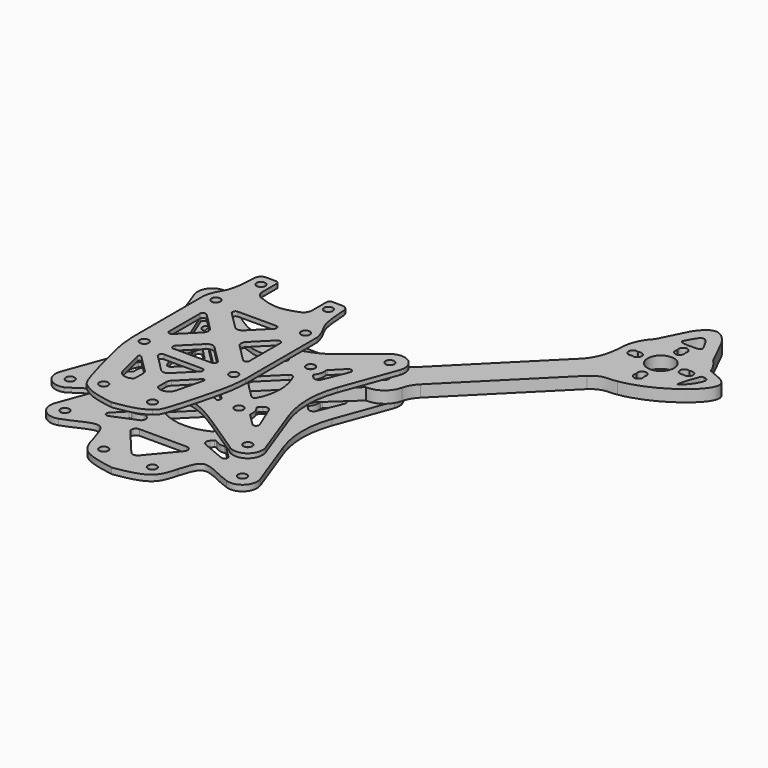
from build123d import *

# Parameters (mm, degrees)
F0_R     = 1.5
F2_DEPTH = 2
F4_START = 3
F1_R     = 1.5
F1_R_2   = 4.5
F4_DEPTH = 4
F7_START = 20
F6_R     = 1.5
F7_DEPTH = 1.5
F8_START = 9
F5_R     = 1.5
F8_DEPTH = 1.5


with BuildPart() as f2:
    # F0 (on Top) → F2 (new body)
    with BuildSketch(Plane.XY):
        with BuildLine():
            add(Edge.make_bspline(
                [(-28.6583371689, 34.989895508), (-15.5486081514, 28.1029236725), (-15.2531134537, 20.3288752095), (-15.0275822655, 35.7869570093)],
                knots=[0, 0, 0, 0, 13.3992828802, 13.3992828802, 13.3992828802, 13.3992828802], degree=3))
            ThreePointArc((-28.6583371689, 34.989895508), (-33.8221162144, 33.7485690999), (-34.9557615497, 28.560086322))
            Line((-34.9557615497, 28.560086322), (-28.2756954338, 10.3133747837))
            ThreePointArc((-28.2756954338, 10.3133747837), (-26.4471685044, -7.1088e-06), (-28.2756201348, -10.3134023513))
            Line((-28.2756201348, -10.3134023513), (-34.9643155344, -28.58409813))
            ThreePointArc((-34.9643155344, -28.58409813), (-33.8042341838, -33.7667341911), (-28.6341939914, -34.9817196608))
            add(Edge.make_bspline(
                [(-28.6341939914, -34.9817196608), (-24.495487875, -33.6930387827), (-16.3607874703, -27.7449542077), (-15.1366587225, -35.7631260416), (-14.33, -37.7577804035)],
                knots=[0, 0, 0, 0, 0.5615113554, 1, 1, 1, 1], degree=3))
            add(Edge.make_bspline(
                [(-14.33, -37.7577804035), (-13.6367446794, -40.3263257967), (-12.088150953, -46.0639424644), (-4.3010614265, -47.3817279873), (0, -48.1095835567)],
                knots=[0, 0, 0, 0, 0.447667654, 1, 1, 1, 1], degree=3))
            add(Edge.make_bspline(
                [(14.33, -37.7577804035), (13.6367446794, -40.3263257967), (12.088150953, -46.0639424644), (4.3010614265, -47.3817279873), (0, -48.1095835567)],
                knots=[0, 0, 0, 0, 0.447667654, 1, 1, 1, 1], degree=3))
            add(Edge.make_bspline(
                [(28.6583371689, -34.9898955092), (24.5097770544, -33.6967999), (16.3601661117, -27.7422129401), (15.1363049951, -35.7630085829), (14.33, -37.7577804035)],
                knots=[0, 0, 0, 0, 0.561784833, 1, 1, 1, 1], degree=3))
            ThreePointArc((28.6583371689, -34.9898955092), (33.8221162144, -33.748569101), (34.9557615497, -28.5600863232))
            Line((34.9557615497, -28.5600863232), (28.2756954338, -10.3133747849))
            ThreePointArc((28.2756954338, -10.3133747849), (26.4471685044, 7.1077e-06), (28.2756201348, 10.3134023502))
            Line((28.2756201348, 10.3134023502), (34.9643155344, 28.5840981288))
            ThreePointArc((34.9643155344, 28.5840981288), (33.8042341838, 33.76673419), (28.6341939914, 34.9817196596))
            add(Edge.make_bspline(
                [(15.0274820378, 35.7867377887), (15.2513136358, 20.3289797995), (15.5248044507, 28.1031931102), (28.6341939914, 34.9817196596)],
                knots=[0.5359060708, 0.5359060708, 0.5359060708, 0.5359060708, 13.9139411757, 13.9139411757, 13.9139411757, 13.9139411757], degree=3))
            ThreePointArc((15.0274820378, 35.7867377887), (14.4316299327, 37.1821951546), (13.0276916813, 37.7577804023))
            Line((13.0276916813, 37.7577804023), (-13.0277950954, 37.7577804023))
            ThreePointArc((-13.0277950954, 37.7577804023), (-14.4316552711, 37.1822721036), (-15.0275822655, 35.7869570093))
        make_face()
        with Locations((-30.25, -30.2500000006)):
            Circle(F0_R, mode=Mode.SUBTRACT)
        with Locations((-8.2733329443, -41.1618490551)):
            Circle(F0_R, mode=Mode.SUBTRACT)
        with BuildLine():
            ThreePointArc((-23.8517090122, -20.3161751069), (-25.1141961389, -20.4406647854), (-25.4828700073, -19.2268068843))
            Line((-25.4828700073, -19.2268068843), (-22.1833207357, -11.2506887671))
            ThreePointArc((-22.1833207357, -11.2506887671), (-21.0902108457, -10.3529698728), (-19.736579243, -10.7634207575))
            Line((-19.736579243, -10.7634207575), (-18.8553009264, -11.6446990741))
            ThreePointArc((-18.8553009264, -11.6446990741), (-18.7090370991, -11.9847340093), (-18.8367068235, -12.33217797))
            Line((-18.8367068235, -12.33217797), (-18.8542943682, -12.3517786311))
            ThreePointArc((-18.8542943682, -12.3517786311), (-19.6877326512, -13.9472514003), (-19.8489637612, -15.7400584892))
            Line((-19.8489637612, -15.7400584892), (-19.8303976916, -15.8549305034))
            ThreePointArc((-19.8303976916, -15.8549305034), (-19.8571321349, -16.2052315209), (-20.0404595752, -16.5049256699))
            Line((-20.0404595752, -16.5049256699), (-23.8517090122, -20.3161751069))
        make_face(mode=Mode.SUBTRACT)
        with BuildLine():
            Line((-11.2506887665, -22.1833207364), (-19.2268068836, -25.482870008))
            ThreePointArc((-19.2268068836, -25.482870008), (-20.4406647847, -25.1141961396), (-20.3161751062, -23.8517090128))
            Line((-20.3161751062, -23.8517090128), (-16.5049256693, -20.0404595759))
            ThreePointArc((-16.5049256693, -20.0404595759), (-16.2052315202, -19.8571321356), (-15.8549305027, -19.8303976923))
            Line((-15.8549305027, -19.8303976923), (-15.7400584885, -19.8489637619))
            ThreePointArc((-15.7400584885, -19.8489637619), (-13.9472513996, -19.6877326519), (-12.3517786304, -18.8542943689))
            Line((-12.3517786304, -18.8542943689), (-12.3321779693, -18.8367068242))
            ThreePointArc((-12.3321779693, -18.8367068242), (-11.9847340086, -18.7090370997), (-11.6446990734, -18.8553009271))
            Line((-11.6446990734, -18.8553009271), (-10.7634207569, -19.7365792436))
            ThreePointArc((-10.7634207569, -19.7365792436), (-10.3529698721, -21.0902108464), (-11.2506887665, -22.1833207364))
        make_face(mode=Mode.SUBTRACT)
        with Locations((-15.25, -15.2500000006)):
            Circle(F0_R, mode=Mode.SUBTRACT)
        with BuildLine():
            ThreePointArc((-7.7892382513, -15.2383616248), (-8.2896410828, -14.5053634666), (-8.0071487762, -13.6640030263))
            Line((-8.0071487762, -13.6640030263), (-1.4142135624, -7.0710678125))
            ThreePointArc((-1.4142135624, -7.0710678125), (0, -6.4852813748), (1.4142135624, -7.0710678125))
            Line((1.4142135624, -7.0710678125), (8.0039929944, -13.6608472445))
            ThreePointArc((8.0039929944, -13.6608472445), (8.287442711, -14.5050591849), (7.7853439372, -15.2405415869))
            Line((7.7853439372, -15.2405415869), (7.7684472975, -15.2500000006))
            ThreePointArc((7.7684472975, -15.2500000006), (0, -17.1146508417), (-7.7684472975, -15.2500000006))
            Line((-7.7684472975, -15.2500000006), (-7.7892382513, -15.2383616248))
        make_face(mode=Mode.SUBTRACT)
        with Locations((8.2733329443, -41.1618490551)):
            Circle(F0_R, mode=Mode.SUBTRACT)
        with BuildLine():
            Line((-1.3419338656, -38.0910861377), (-9.1892168108, -28.7161126104))
            ThreePointArc((-9.1892168108, -28.7161126104), (-9.3980668278, -27.118570832), (-8.0389877832, -26.2533181443))
            Line((-8.0389877832, -26.2533181443), (8.0389877833, -26.2533181443))
            ThreePointArc((8.0389877833, -26.2533181443), (9.398066828, -27.118570832), (9.189216811, -28.7161126104))
            Line((9.189216811, -28.7161126104), (1.3419338656, -38.0910861377))
            ThreePointArc((1.3419338656, -38.0910861377), (0, -38.7178259272), (-1.3419338656, -38.0910861377))
        make_face(mode=Mode.SUBTRACT)
        with Locations((30.25, -30.2500000006)):
            Circle(F0_R, mode=Mode.SUBTRACT)
        with BuildLine():
            ThreePointArc((20.3161751064, -23.8517090128), (20.4406647849, -25.1141961396), (19.2268068838, -25.482870008))
            Line((19.2268068838, -25.482870008), (11.2506887667, -22.1833207364))
            ThreePointArc((11.2506887667, -22.1833207364), (10.3529698723, -21.0902108464), (10.7634207571, -19.7365792436))
            Line((10.7634207571, -19.7365792436), (11.6446990736, -18.8553009271))
            ThreePointArc((11.6446990736, -18.8553009271), (11.9847340088, -18.7090370997), (12.3321779695, -18.8367068242))
            Line((12.3321779695, -18.8367068242), (12.3517786306, -18.8542943689))
            ThreePointArc((12.3517786306, -18.8542943689), (13.9472513998, -19.6877326519), (15.7400584887, -19.8489637619))
            Line((15.7400584887, -19.8489637619), (15.8549305029, -19.8303976923))
            ThreePointArc((15.8549305029, -19.8303976923), (16.2052315204, -19.8571321356), (16.5049256694, -20.0404595759))
            Line((16.5049256694, -20.0404595759), (20.3161751064, -23.8517090128))
        make_face(mode=Mode.SUBTRACT)
        with Locations((15.25, -15.2500000006)):
            Circle(F0_R, mode=Mode.SUBTRACT)
        with BuildLine():
            ThreePointArc((19.7365792431, -10.7634207575), (21.0902108459, -10.3529698728), (22.1833207359, -11.2506887671))
            Line((22.1833207359, -11.2506887671), (25.4828700075, -19.2268068842))
            ThreePointArc((25.4828700075, -19.2268068842), (25.1141961391, -20.4406647853), (23.8517090123, -20.3161751069))
            Line((23.8517090123, -20.3161751069), (20.0404595754, -16.5049256699))
            ThreePointArc((20.0404595754, -16.5049256699), (19.8571321351, -16.2052315209), (19.8303976918, -15.8549305033))
            Line((19.8303976918, -15.8549305033), (19.8489637614, -15.7400584892))
            ThreePointArc((19.8489637614, -15.7400584892), (19.6877326514, -13.9472514003), (18.8542943684, -12.3517786311))
            Line((18.8542943684, -12.3517786311), (18.8367068237, -12.33217797))
            ThreePointArc((18.8367068237, -12.33217797), (18.7090370992, -11.9847340093), (18.8553009266, -11.6446990741))
            Line((18.8553009266, -11.6446990741), (19.7365792431, -10.7634207575))
        make_face(mode=Mode.SUBTRACT)
        with BuildLine():
            ThreePointArc((-18.8367068237, 12.3321779688), (-18.7090370992, 11.9847340081), (-18.8553009266, 11.6446990729))
            Line((-18.8553009266, 11.6446990729), (-19.7365318181, 10.7634681813))
            ThreePointArc((-19.7365318181, 10.7634681813), (-21.0901735727, 10.3530193183), (-22.1832812244, 11.250755321))
            Line((-22.1832812244, 11.250755321), (-25.4825410679, 19.2264854211))
            ThreePointArc((-25.4825410679, 19.2264854211), (-25.1138561851, 20.4403344014), (-23.851374797, 20.3158408904))
            Line((-23.851374797, 20.3158408904), (-20.0404595754, 16.5049256687))
            ThreePointArc((-20.0404595754, 16.5049256687), (-19.8571321351, 16.2052315197), (-19.8303976918, 15.8549305022))
            Line((-19.8303976918, 15.8549305022), (-19.8489637614, 15.740058488))
            ThreePointArc((-19.8489637614, 15.740058488), (-19.6877326514, 13.9472513991), (-18.8542943684, 12.3517786299))
            Line((-18.8542943684, 12.3517786299), (-18.8367068237, 12.3321779688))
        make_face(mode=Mode.SUBTRACT)
        with BuildLine():
            ThreePointArc((-13.6608472446, -8.003992994), (-14.505059185, -8.2874427105), (-15.2405415869, -7.7853439367))
            Line((-15.2405415869, -7.7853439367), (-15.25, -7.7684472983))
            ThreePointArc((-15.25, -7.7684472983), (-17.1146508411, -6e-10), (-15.25, 7.7684472971))
            Line((-15.25, 7.7684472971), (-15.2405415859, 7.7853439372))
            ThreePointArc((-15.2405415859, 7.7853439372), (-14.505059184, 8.2874427111), (-13.6608472436, 8.0039929945))
            Line((-13.6608472436, 8.0039929945), (-7.0710678122, 1.4142135631))
            ThreePointArc((-7.0710678122, 1.4142135631), (-6.4852813746, 7e-10), (-7.0710678122, -1.4142135616))
            Line((-7.0710678122, -1.4142135616), (-13.6608472446, -8.003992994))
        make_face(mode=Mode.SUBTRACT)
        with Locations((-15.25, 15.2499999994)):
            Circle(F0_R, mode=Mode.SUBTRACT)
        with BuildLine():
            ThreePointArc((7.7853439372, 15.2405415857), (8.287442711, 14.5050591838), (8.0039929944, 13.6608472433))
            Line((8.0039929944, 13.6608472433), (1.4142135624, 7.0710678113))
            ThreePointArc((1.4142135624, 7.0710678113), (0, 6.4852813737), (-1.4142135624, 7.0710678113))
            Line((-1.4142135624, 7.0710678113), (-8.0039929944, 13.6608472433))
            ThreePointArc((-8.0039929944, 13.6608472433), (-8.287442711, 14.5050591838), (-7.7853439372, 15.2405415857))
            Line((-7.7853439372, 15.2405415857), (-7.7684472975, 15.2499999994))
            ThreePointArc((-7.7684472975, 15.2499999994), (0, 17.1146508406), (7.7684472975, 15.2499999994))
            Line((7.7684472975, 15.2499999994), (7.7853439372, 15.2405415857))
        make_face(mode=Mode.SUBTRACT)
        with Locations((-30.25, 30.2499999994)):
            Circle(F0_R, mode=Mode.SUBTRACT)
        with BuildLine():
            ThreePointArc((-7.7684472975, 20.1190513336), (-9.4080907996, 20.7386520685), (-8.9382902045, 22.4273270773))
            Line((-8.9382902045, 22.4273270773), (-1.06072927, 27.355528746))
            ThreePointArc((-1.06072927, 27.355528746), (0, 27.6599894761), (1.0607292699, 27.355528746))
            Line((1.0607292699, 27.355528746), (8.9382902045, 22.4273270773))
            ThreePointArc((8.9382902045, 22.4273270773), (9.4121452662, 20.7467816187), (7.7853439372, 20.1125189809))
            ThreePointArc((7.7853439372, 20.1125189809), (0.0090577048, 21.5667549236), (-7.7684472975, 20.1190513336))
        make_face(mode=Mode.SUBTRACT)
        with Locations((-11.5, 29.7577804023)):
            Circle(F0_R, mode=Mode.SUBTRACT)
        with BuildLine():
            Line((7.0710678124, 1.4142135624), (13.6608472439, 8.0039929938))
            ThreePointArc((13.6608472439, 8.0039929938), (14.5050591843, 8.2874427104), (15.2405415863, 7.7853439366))
            Line((15.2405415863, 7.7853439366), (15.25, 7.7684472971))
            ThreePointArc((15.25, 7.7684472971), (17.1146508411, -6e-10), (15.25, -7.7684472983))
            Line((15.25, -7.7684472983), (15.2405415867, -7.7853439371))
            ThreePointArc((15.2405415867, -7.7853439371), (14.5050591848, -8.2874427109), (13.6608472444, -8.0039929943))
            Line((13.6608472444, -8.0039929943), (7.0710678124, -1.4142135624))
            ThreePointArc((7.0710678124, -1.4142135624), (6.4852813748, 0), (7.0710678124, 1.4142135624))
        make_face(mode=Mode.SUBTRACT)
        with Locations((15.25, 15.2499999994)):
            Circle(F0_R, mode=Mode.SUBTRACT)
        with BuildLine():
            Line((19.8247048971, 15.785759925), (19.8053184489, 15.9004963368))
            ThreePointArc((19.8053184489, 15.9004963368), (19.8295490283, 16.2509794496), (20.0107302331, 16.5519759685))
            Line((20.0107302331, 16.5519759685), (23.8084562188, 20.4043695836))
            ThreePointArc((23.8084562188, 20.4043695836), (25.0693920791, 20.5382911332), (25.4479247727, 19.3280815542))
            Line((25.4479247727, 19.3280815542), (22.2099579078, 11.3050038785))
            ThreePointArc((22.2099579078, 11.3050038785), (21.1235499455, 10.3976310998), (19.7659136105, 10.7981697397))
            Line((19.7659136105, 10.7981697397), (18.8636878016, 11.6875924575))
            ThreePointArc((18.8636878016, 11.6875924575), (18.7150078324, 12.0262851571), (18.8397994936, 12.37448843))
            Line((18.8397994936, 12.37448843), (18.8575858105, 12.3946446988))
            ThreePointArc((18.8575858105, 12.3946446988), (19.6770217108, 13.9944130467), (19.8247048971, 15.785759925))
        make_face(mode=Mode.SUBTRACT)
        with Locations((11.5, 29.7577804023)):
            Circle(F0_R, mode=Mode.SUBTRACT)
        with Locations((30.25, 30.2499999994)):
            Circle(F0_R, mode=Mode.SUBTRACT)
    extrude(amount=F2_DEPTH)


with BuildPart() as f4:
    # F1 (on Top) → F4 (new body)
    with BuildSketch(Plane.XY.offset(F4_START)):
        with BuildLine():
            add(Edge.make_bspline(
                [(77.2593953395, 101.7986398484), (78.7593953395, 104.1420138718), (82.5093953395, 107.8579861282), (86.2593953395, 104.1420138718), (87.7593953395, 101.7986398484)],
                knots=[0, 0, 0, 0, 0.5, 1, 1, 1, 1], degree=3))
            Line((77.2593953395, 101.7986398484), (72.6099004029, 92.3994949366))
            ThreePointArc((72.6099004029, 92.3994949366), (69.5750818843, 87.8575680531), (68.5093953395, 82.5))
            add(Edge.make_bspline(
                [(64.6217106464, 71.6833831188), (67.2594552161, 74.6181810973), (68.3412179351, 78.679420054), (68.5093953395, 82.5)],
                knots=[0, 0, 0, 0, 11.4940546817, 11.4940546817, 11.4940546817, 11.4940546817], degree=3))
            Line((64.6217106464, 71.6833831188), (33.0976358255, 40.1593082979))
            ThreePointArc((33.0976358255, 40.1593082979), (30.9505970873, 38.5267023061), (28.4453264856, 37.5273040471))
            ThreePointArc((28.4453264856, 37.5273040471), (24.6916297412, 35.2749364416), (22.834774137, 31.3106601718))
            Line((22.834774137, 31.3106601718), (13.6185183249, 19.9730840161))
            ThreePointArc((13.6185183249, 19.9730840161), (11.3998018999, 18.428606374), (10.3093393921, 15.9549440526))
            Line((10.3093393921, 15.9549440526), (6.3693953395, 12.015))
            Line((6.3693953395, 12.015), (0.0093953395, 5.655))
            Line((0.0093953395, 5.655), (0.0093953395, 0))
            Line((0.0093953395, 0), (5.6643953395, 0))
            Line((5.6643953395, 0), (12.0243953395, 6.36))
            Line((12.0243953395, 6.36), (15.964339392, 10.2999440526))
            ThreePointArc((15.964339392, 10.2999440526), (18.4380017135, 11.3904065604), (19.9824793556, 13.6091229854))
            Line((19.9824793556, 13.6091229854), (29.8420821702, 22.7616190189))
            ThreePointArc((29.8420821702, 22.7616190189), (34.7107235952, 24.2138027898), (37.5366993865, 28.4359311461))
            ThreePointArc((37.5366993865, 28.4359311461), (38.5360976455, 30.9412017478), (40.1687036374, 33.0882404861))
            Line((40.1687036374, 33.0882404861), (71.6788756749, 64.5984125236))
            add(Edge.make_bspline(
                [(71.6788756749, 64.5984125236), (75.2138197422, 67.773707211), (77.5027647614, 66.6008293629), (80.0291356677, 67.1997283697)],
                knots=[0, 0, 0, 0, 8.7460668919, 8.7460668919, 8.7460668919, 8.7460668919], degree=3))
            add(Edge.make_bspline(
                [(95.6294447875, 87.3851102834), (98.5490253606, 86.1806662064), (109.349192454, 82.9975524374), (90.7150401258, 68.8518105531), (80.0291356677, 67.1997283697)],
                knots=[0, 0, 0, 0, 0.3577567319, 1, 1, 1, 1], degree=3))
            ThreePointArc((95.6294447875, 87.3851102834), (94.2890756952, 90.0656546787), (92.4088902761, 92.3994949366))
            Line((92.4088902761, 92.3994949366), (87.7593953395, 101.7986398484))
        make_face()
        with Locations((15.2593953395, 15.25)):
            Circle(F1_R, mode=Mode.SUBTRACT)
        with Locations((30.2593953395, 30.25)):
            Circle(F1_R, mode=Mode.SUBTRACT)
        with BuildLine():
            ThreePointArc((83.8084334452, 73.75), (82.5093953395, 71.5), (81.2103572338, 73.75))
            ThreePointArc((81.2103572338, 73.75), (82.5093953395, 76), (83.8084334452, 73.75))
        make_face(mode=Mode.SUBTRACT)
        with BuildLine():
            add(Edge.make_bspline(
                [(96.4851732404, 83.323184101), (95.8861932158, 83.3624526858), (95.6489634201, 83.406211956), (92.4634486437, 74.1656348109), (94.1752940416, 76.0721862316)],
                knots=[0, 0, 0, 0, 0.3095337058, 1, 1, 1, 1], degree=3))
            add(Edge.make_bspline(
                [(96.4851732404, 83.323184101), (97.1968024969, 83.2540988922), (99.2072247022, 82.7650440123), (96.5406354296, 78.1400697337), (94.1752940416, 76.0721862316)],
                knots=[0, 0, 0, 0, 0.324824519, 1, 1, 1, 1], degree=3))
        make_face(mode=Mode.SUBTRACT)
        with BuildLine():
            ThreePointArc((73.7593953395, 83.7990381057), (76.0093953395, 82.5), (73.7593953395, 81.2009618943))
            ThreePointArc((73.7593953395, 81.2009618943), (71.5093953395, 82.5), (73.7593953395, 83.7990381057))
        make_face(mode=Mode.SUBTRACT)
        with Locations((82.5093953395, 82.5)):
            Circle(F1_R_2, mode=Mode.SUBTRACT)
        with BuildLine():
            ThreePointArc((91.2593953395, 81.2009618943), (89.0093953395, 82.5), (91.2593953395, 83.7990381057))
            ThreePointArc((91.2593953395, 83.7990381057), (93.5093953395, 82.5), (91.2593953395, 81.2009618943))
        make_face(mode=Mode.SUBTRACT)
        with BuildLine():
            ThreePointArc((83.8084334452, 91.25), (82.5093953395, 89), (81.2103572338, 91.25))
            ThreePointArc((81.2103572338, 91.25), (82.5093953395, 93.5), (83.8084334452, 91.25))
        make_face(mode=Mode.SUBTRACT)
        with BuildLine():
            add(Edge.make_bspline(
                [(79.0163052703, 96.0572239698), (79.135660109, 95.064372308), (82.5093953395, 95.064372308), (85.88313057, 95.064372308), (86.0024854087, 96.0572239698)],
                knots=[0, 0, 0, 0, 0.5, 1, 1, 1, 1], degree=3))
            add(Edge.make_bspline(
                [(79.0163052703, 96.0572239698), (80.1806686267, 98.4065499989), (82.5093953395, 103.1052020569), (84.8381220523, 98.4065499989), (86.0024854087, 96.0572239698)],
                knots=[0, 0, 0, 0, 0.5, 1, 1, 1, 1], degree=3))
        make_face(mode=Mode.SUBTRACT)
    extrude(amount=F4_DEPTH)


with BuildPart() as f7:
    # F6 (on Top) → F7 (new body)
    with BuildSketch(Plane.XY.offset(F7_START)):
        with BuildLine():
            add(Edge.make_bspline(
                [(-19.25, -15.2218541075), (-19.0684905374, -19.7268529833), (-17.9623264747, -24.6907042809), (-13.2785718821, -43.084666195), (-11.6053951728, -44.1968771124), (-11.0003547743, -44.5749795424)],
                knots=[0, 0, 0, 0, 0.3683029461, 0.8298524693, 1, 1, 1, 1], degree=3))
            add(Edge.make_bspline(
                [(-11.0003547743, -44.5749795424), (-7.8986920416, -46.9837644324), (-3.9995196275, -47.3454079802), (0, -48.1093942399)],
                knots=[0, 0, 0, 0, 11.5542153526, 11.5542153526, 11.5542153526, 11.5542153526], degree=3))
            add(Edge.make_bspline(
                [(11.0003547743, -44.5749795424), (7.8986920416, -46.9837644324), (3.9995196275, -47.3454079802), (0, -48.1093942399)],
                knots=[0, 0, 0, 0, 11.5542153526, 11.5542153526, 11.5542153526, 11.5542153526], degree=3))
            add(Edge.make_bspline(
                [(19.25, -15.2218541075), (19.0667337669, -19.7267716154), (17.9562925595, -24.6902276301), (13.2790290127, -43.0847539077), (11.6055152346, -44.1969091306), (11.0003547743, -44.5749795424)],
                knots=[0, 0, 0, 0, 0.368314136, 0.829851714, 1, 1, 1, 1], degree=3))
            Line((19.25, -15.2218541075), (19.25, 15.2781458925))
            add(Edge.make_bspline(
                [(15.0790967662, 31.8597836794), (15.7273210805, 18.4148469189), (17.670676786, 22.4575338068), (19.25, 15.2781458925)],
                knots=[0.8128411452, 0.8128411452, 0.8128411452, 0.8128411452, 18.97635654, 18.97635654, 18.97635654, 18.97635654], degree=3))
            ThreePointArc((15.0790967662, 31.8597836794), (14.4611582834, 33.211334576), (13.0814172406, 33.7634690247))
            add(Edge.make_bspline(
                [(9.5020394819, 33.7713114856), (10.6902314797, 33.7688881845), (11.9558724743, 33.7634690247), (13.0814172406, 33.7634690247)],
                knots=[1.0243447025, 1.0243447025, 1.0243447025, 1.0243447025, 4.5814260604, 4.5814260604, 4.5814260604, 4.5814260604], degree=3))
            ThreePointArc((9.5020394819, 33.7713114856), (8.7936146526, 33.479141045), (8.5, 32.7713135654))
            add(Edge.make_bspline(
                [(8.5, 32.285449478), (8.5, 32.4472244474), (8.5, 32.609243629), (8.5, 32.7713135654)],
                knots=[0.2605482636, 0.2605482636, 0.2605482636, 0.2605482636, 0.7461719983, 0.7461719983, 0.7461719983, 0.7461719983], degree=3))
            add(Edge.make_bspline(
                [(8.5, 32.025302314), (8.5, 32.1119278185), (8.5, 32.1986534992), (8.5, 32.285449478)],
                knots=[0, 0, 0, 0, 0.2605482636, 0.2605482636, 0.2605482636, 0.2605482636], degree=3))
            Line((8.5, 32.025302314), (8.5, 26.5908181775))
            ThreePointArc((8.5, 26.5908181775), (7.9671627129, 24.8840351954), (6.5579279014, 23.7835439559))
            add(Edge.make_bspline(
                [(-6.5579279014, 23.7835439559), (-4.3358517051, 22.9461493085), (0, 21.578151535), (4.3358517051, 22.9461493085), (6.5579279014, 23.7835439559)],
                knots=[0.1121315865, 0.1121315865, 0.1121315865, 0.1121315865, 0.5, 0.8878684135, 0.8878684135, 0.8878684135, 0.8878684135], degree=3))
            ThreePointArc((-6.5579279014, 23.7835439559), (-7.9671627129, 24.8840351954), (-8.5, 26.5908181775))
            Line((-8.5, 26.5908181775), (-8.5, 32.025302314))
            add(Edge.make_bspline(
                [(-8.5, 32.025302314), (-8.5, 32.1119278185), (-8.5, 32.1986534992), (-8.5, 32.285449478)],
                knots=[0, 0, 0, 0, 0.2605482636, 0.2605482636, 0.2605482636, 0.2605482636], degree=3))
            add(Edge.make_bspline(
                [(-8.5, 32.285449478), (-8.5, 32.4469519552), (-8.5, 32.6086978226), (-8.5, 32.7704945986)],
                knots=[0.2605482636, 0.2605482636, 0.2605482636, 0.2605482636, 0.7453540183, 0.7453540183, 0.7453540183, 0.7453540183], degree=3))
            ThreePointArc((-8.5, 32.7704945986), (-8.7935873047, 33.4782947851), (-9.501962208, 33.7704926735))
            Line((-9.501962208, 33.7704926735), (-13.0814172406, 33.7634690247))
            ThreePointArc((-13.0814172406, 33.7634690247), (-14.4611582834, 33.211334576), (-15.0790967662, 31.8597836794))
            add(Edge.make_bspline(
                [(-15.0790967662, 31.8597836794), (-15.7273210805, 18.4148469189), (-17.670676786, 22.4575338068), (-19.25, 15.2781458925)],
                knots=[0.8128411452, 0.8128411452, 0.8128411452, 0.8128411452, 18.97635654, 18.97635654, 18.97635654, 18.97635654], degree=3))
            Line((-19.25, 15.2781458925), (-19.25, -15.2218541075))
        make_face()
        with Locations((-8.3293477558, -41.1257331912)):
            Circle(F6_R, mode=Mode.SUBTRACT)
        with BuildLine():
            ThreePointArc((-11.2741795299, -22.9536277928), (-11.0338873267, -22.3989447209), (-10.4349964383, -22.4810626653))
            Line((-10.4349964383, -22.4810626653), (-4.5076118446, -28.408447259))
            ThreePointArc((-4.5076118446, -28.408447259), (-4.0740663419, -29.0572939567), (-3.9218254069, -29.8226608214))
            Line((-3.9218254069, -29.8226608214), (-3.9218254069, -32.9968597055))
            ThreePointArc((-3.9218254069, -32.9968597055), (-4.0264596985, -33.4421913215), (-4.3184659033, -33.7943290211))
            Line((-4.3184659033, -33.7943290211), (-4.4003069963, -33.8562493989))
            ThreePointArc((-4.4003069963, -33.8562493989), (-7.223873087, -34.0855754205), (-9.0722171951, -31.9387778169))
            Line((-9.0722171951, -31.9387778169), (-11.2741795299, -22.9536277928))
        make_face(mode=Mode.SUBTRACT)
        with Locations((-15.25, -15.2218541075)):
            Circle(F6_R, mode=Mode.SUBTRACT)
        with Locations((8.3288047093, -41.1259644251)):
            Circle(F6_R, mode=Mode.SUBTRACT)
        with BuildLine():
            Line((4.5076118446, -28.408447259), (10.4349123369, -22.4811467667))
            ThreePointArc((10.4349123369, -22.4811467667), (11.0338107336, -22.3990330505), (11.2740913261, -22.9537286326))
            Line((11.2740913261, -22.9537286326), (9.0718254069, -31.9387778169))
            ThreePointArc((9.0718254069, -31.9387778169), (7.2237469097, -34.0856955052), (4.4002690575, -33.8562995378))
            Line((4.4002690575, -33.8562995378), (4.3183823385, -33.7943311455))
            ThreePointArc((4.3183823385, -33.7943311455), (4.0264363662, -33.4422097633), (3.9218254069, -32.9969250614))
            Line((3.9218254069, -32.9969250614), (3.9218254069, -29.8226608214))
            ThreePointArc((3.9218254069, -29.8226608214), (4.0740663419, -29.0572939567), (4.5076118446, -28.408447259))
        make_face(mode=Mode.SUBTRACT)
        with BuildLine():
            Line((-1.4142135624, -25.3091152098), (-7.2178932188, -19.5054355534))
            ThreePointArc((-7.2178932188, -19.5054355534), (-7.4346659701, -18.4156453398), (-6.5107864376, -17.7983287722))
            Line((-6.5107864376, -17.7983287722), (6.5107864376, -17.7983287722))
            ThreePointArc((6.5107864376, -17.7983287722), (7.4346659701, -18.4156453398), (7.2178932188, -19.5054355534))
            Line((7.2178932188, -19.5054355534), (1.4142135624, -25.3091152098))
            ThreePointArc((1.4142135624, -25.3091152098), (0, -25.8949016474), (-1.4142135624, -25.3091152098))
        make_face(mode=Mode.SUBTRACT)
        with BuildLine():
            ThreePointArc((-1.4142135624, -6.1360676699), (0, -5.5502812323), (1.4142135624, -6.1360676699))
            Line((1.4142135624, -6.1360676699), (7.2178932188, -11.9397473263))
            ThreePointArc((7.2178932188, -11.9397473263), (7.4346659701, -13.0295375399), (6.5107864376, -13.6468541075))
            Line((6.5107864376, -13.6468541075), (-6.5107864376, -13.6468541075))
            ThreePointArc((-6.5107864376, -13.6468541075), (-7.4346659701, -13.0295375399), (-7.2178932188, -11.9397473263))
            Line((-7.2178932188, -11.9397473263), (-1.4142135624, -6.1360676699))
        make_face(mode=Mode.SUBTRACT)
        with Locations((15.25, -15.2218541075)):
            Circle(F6_R, mode=Mode.SUBTRACT)
        with BuildLine():
            Line((-11.9678932188, 7.2460391113), (-6.1642135624, 1.4423594549))
            ThreePointArc((-6.1642135624, 1.4423594549), (-5.5784271247, 0.0281458925), (-6.1642135624, -1.3860676699))
            Line((-6.1642135624, -1.3860676699), (-11.9678932188, -7.1897473263))
            ThreePointArc((-11.9678932188, -7.1897473263), (-13.0576834324, -7.4065200777), (-13.675, -6.4826405451))
            Line((-13.675, -6.4826405451), (-13.675, 6.5389323301))
            ThreePointArc((-13.675, 6.5389323301), (-13.0576834324, 7.4628118626), (-11.9678932188, 7.2460391113))
        make_face(mode=Mode.SUBTRACT)
        with Locations((-15.25, 15.2781458925)):
            Circle(F6_R, mode=Mode.SUBTRACT)
        with Locations((-11.499689569, 29.7634854823)):
            Circle(F6_R, mode=Mode.SUBTRACT)
        with BuildLine():
            ThreePointArc((1.4142135624, 6.1923594549), (0, 5.6065730172), (-1.4142135624, 6.1923594549))
            Line((-1.4142135624, 6.1923594549), (-7.2178932188, 11.9960391113))
            ThreePointArc((-7.2178932188, 11.9960391113), (-7.4346659701, 13.0858293249), (-6.5107864376, 13.7031458925))
            Line((-6.5107864376, 13.7031458925), (6.5107864376, 13.7031458925))
            ThreePointArc((6.5107864376, 13.7031458925), (7.4346659701, 13.0858293249), (7.2178932188, 11.9960391113))
            Line((7.2178932188, 11.9960391113), (1.4142135624, 6.1923594549))
        make_face(mode=Mode.SUBTRACT)
        with BuildLine():
            Line((11.9678932188, -7.1897473263), (6.1642135624, -1.3860676699))
            ThreePointArc((6.1642135624, -1.3860676699), (5.5784271247, 0.0281458925), (6.1642135624, 1.4423594549))
            Line((6.1642135624, 1.4423594549), (11.9678932188, 7.2460391113))
            ThreePointArc((11.9678932188, 7.2460391113), (13.0576834324, 7.4628118626), (13.675, 6.5389323301))
            Line((13.675, 6.5389323301), (13.675, -6.4826405451))
            ThreePointArc((13.675, -6.4826405451), (13.0576834324, -7.4065200777), (11.9678932188, -7.1897473263))
        make_face(mode=Mode.SUBTRACT)
        with Locations((15.25, 15.2781458925)):
            Circle(F6_R, mode=Mode.SUBTRACT)
        with Locations((11.499689569, 29.7634854822)):
            Circle(F6_R, mode=Mode.SUBTRACT)
    extrude(amount=F7_DEPTH)


with BuildPart() as f8:
    # F5 (on Top) → F8 (new body)
    with BuildSketch(Plane.XY.offset(F8_START)):
        with BuildLine():
            ThreePointArc((-26.9407032856, 36.2600348998), (-27.7551557637, 36.8489935616), (-28.6709446924, 37.2631623465))
            ThreePointArc((-28.6709446924, 37.2631623465), (-33.8348197995, 36.0222356117), (-34.9688667131, 30.8338405921))
            Line((-34.9688667131, 30.8338405921), (-28.2886697962, 12.5867673035))
            ThreePointArc((-28.2886697962, 12.5867673035), (-26.4601436815, 2.2733832229), (-28.2885975317, -8.0400136697))
            Line((-28.2885975317, -8.0400136697), (-34.9770950156, -26.3101566446))
            ThreePointArc((-34.9770950156, -26.3101566446), (-33.8176199057, -31.4929283694), (-28.6477218702, -32.7085185901))
            ThreePointArc((-28.6477218702, -32.7085185901), (-27.7339748711, -32.2898641192), (-26.9224202046, -31.6969187864))
            Line((-26.9224202046, -31.6969187864), (-15.2629743804, -23.98008234))
            add(Edge.make_bspline(
                [(-15.2629743804, -23.98008234), (-10.179641047, -20.7141435083), (-0.0129743803, -14.1822658449), (10.1536922863, -20.7141435083), (15.2370256196, -23.98008234)],
                knots=[0, 0, 0, 0, 0.5, 1, 1, 1, 1], degree=3))
            Line((15.2370256196, -23.98008234), (26.9147545249, -31.7132548104))
            ThreePointArc((26.9147545249, -31.7132548104), (27.7292070029, -32.3022134723), (28.6449959317, -32.7163822571))
            ThreePointArc((28.6449959317, -32.7163822571), (33.8088710387, -31.4754555224), (34.9429179524, -26.2870605027))
            Line((34.9429179524, -26.2870605027), (28.2627210354, -8.0399872141))
            ThreePointArc((28.2627210354, -8.0399872141), (26.4341949208, 2.2733968665), (28.2626487709, 12.586793759))
            Line((28.2626487709, 12.586793759), (34.9511462548, 30.8569367339))
            ThreePointArc((34.9511462548, 30.8569367339), (33.7916711449, 36.0397084588), (28.6217731094, 37.2552986795))
            ThreePointArc((28.6217731094, 37.2552986795), (27.7080261104, 36.8366442085), (26.8964714439, 36.2436988758))
            Line((26.8964714439, 36.2436988758), (15.2212491446, 26.7733900447))
            add(Edge.make_bspline(
                [(-15.2787508554, 26.7733900447), (-10.8797858751, 23.8265282552), (-0.0532688862, 20.1720392091), (10.8797858751, 23.8112762216), (15.2212491446, 26.7733900447)],
                knots=[0, 0, 0, 0, 0.5000467941, 1, 1, 1, 1], degree=3))
            Line((-15.2787508554, 26.7733900447), (-26.9407032856, 36.2600348998))
        make_face()
        with Locations((-30.2629743804, -27.9766099553)):
            Circle(F5_R, mode=Mode.SUBTRACT)
        with BuildLine():
            ThreePointArc((-23.8489069176, -18.0427905908), (-25.1113940444, -18.1672802692), (-25.4800679128, -16.9534223681))
            Line((-25.4800679128, -16.9534223681), (-22.1805186412, -8.977304251))
            ThreePointArc((-22.1805186412, -8.977304251), (-21.0874087512, -8.0795853567), (-19.7337771484, -8.4900362414))
            Line((-19.7337771484, -8.4900362414), (-18.8524988319, -9.3713145579))
            ThreePointArc((-18.8524988319, -9.3713145579), (-18.7062350045, -9.7113494932), (-18.833904729, -10.0587934538))
            Line((-18.833904729, -10.0587934538), (-18.8514922737, -10.0783941149))
            ThreePointArc((-18.8514922737, -10.0783941149), (-19.6849305567, -11.6738668841), (-19.8461616667, -13.466673973))
            Line((-19.8461616667, -13.466673973), (-19.8275955971, -13.5815459872))
            ThreePointArc((-19.8275955971, -13.5815459872), (-19.8543300404, -13.9318470047), (-20.0376574807, -14.2315411538))
            Line((-20.0376574807, -14.2315411538), (-23.8489069176, -18.0427905908))
        make_face(mode=Mode.SUBTRACT)
        with Locations((-15.2471979054, -12.9766154845)):
            Circle(F5_R, mode=Mode.SUBTRACT)
        with BuildLine():
            ThreePointArc((-13.6600131315, -5.726668306), (-14.5041657047, -6.0102947774), (-15.2397532199, -5.5083500098))
            Line((-15.2397532199, -5.5083500098), (-15.2471979054, -5.4950572526))
            ThreePointArc((-15.2471979054, -5.4950572526), (-17.1135691016, 2.2733900447), (-15.2471979054, 10.041837342))
            Line((-15.2471979054, 10.041837342), (-15.24273859, 10.0498062874))
            ThreePointArc((-15.24273859, 10.0498062874), (-14.5073304159, 10.552013774), (-13.6630765854, 10.2686888511))
            Line((-13.6630765854, 10.2686888511), (-7.0780798423, 3.683692108))
            ThreePointArc((-7.0780798423, 3.683692108), (-6.4922934046, 2.2694785456), (-7.0780798423, 0.8552649832))
            Line((-7.0780798423, 0.8552649832), (-13.6600131315, -5.726668306))
        make_face(mode=Mode.SUBTRACT)
        with Locations((30.2370256196, -27.9766099553)):
            Circle(F5_R, mode=Mode.SUBTRACT)
        with BuildLine():
            ThreePointArc((-7.7816537569, -12.9591669623), (-8.2829493322, -12.2265343934), (-8.001034186, -11.3847674512))
            Line((-8.001034186, -11.3847674512), (-1.427727924, -4.8034136383))
            ThreePointArc((-1.427727924, -4.8034136383), (-0.0138729894, -4.2167621451), (1.4006986714, -4.801683308))
            Line((1.4006986714, -4.801683308), (7.9815684526, -11.37450613))
            ThreePointArc((7.9815684526, -11.37450613), (8.2654849902, -12.2193895506), (7.7626098224, -12.9552925065))
            Line((7.7626098224, -12.9552925065), (7.7244458087, -12.9766154845))
            add(Edge.make_bspline(
                [(-7.7503945694, -12.9766154845), (-5.1645959639, -11.9759777802), (0.0020637685, -9.9766130491), (5.1519589479, -11.9772519711), (7.7244458087, -12.9766154845)],
                knots=[0, 0, 0, 0, 0.5004778212, 1, 1, 1, 1], degree=3))
            Line((-7.7503945694, -12.9766154845), (-7.7816537569, -12.9591669623))
        make_face(mode=Mode.SUBTRACT)
        with Locations((15.2528020946, -12.9766154845)):
            Circle(F5_R, mode=Mode.SUBTRACT)
        with BuildLine():
            Line((7.0557704686, 3.6852806441), (13.6380885864, 10.267598762))
            ThreePointArc((13.6380885864, 10.267598762), (14.4819467408, 10.5509556529), (15.2171693716, 10.0491236138))
            Line((15.2171693716, 10.0491236138), (15.2212491446, 10.041837342))
            ThreePointArc((15.2212491446, 10.041837342), (17.0876203409, 2.2733900447), (15.2212491446, -5.4950572526))
            Line((15.2212491446, -5.4950572526), (15.2156406206, -5.5050714767))
            ThreePointArc((15.2156406206, -5.5050714767), (14.4802031371, -6.0069702904), (13.6361480691, -5.7235240811))
            Line((13.6361480691, -5.7235240811), (7.0557704686, 0.8568535194))
            ThreePointArc((7.0557704686, 0.8568535194), (6.4699840309, 2.2710670817), (7.0557704686, 3.6852806441))
        make_face(mode=Mode.SUBTRACT)
        with BuildLine():
            ThreePointArc((19.7370620173, -8.4877181194), (21.0904813131, -8.0765677155), (22.1840550096, -8.9737215569))
            Line((22.1840550096, -8.9737215569), (25.4877259998, -16.9481333598))
            ThreePointArc((25.4877259998, -16.9481333598), (25.1196795178, -18.1621816342), (23.8571282218, -18.0383444417))
            Line((23.8571282218, -18.0383444417), (20.0439095917, -14.2290652158))
            ThreePointArc((20.0439095917, -14.2290652158), (19.8604272901, -13.9294658528), (19.8335118104, -13.5791786987))
            Line((19.8335118104, -13.5791786987), (19.8520185102, -13.4642971047))
            ThreePointArc((19.8520185102, -13.4642971047), (19.6898608763, -11.6715735815), (18.855598144, -10.0765317569))
            Line((18.855598144, -10.0765317569), (18.8380004718, -10.0569401879))
            ThreePointArc((18.8380004718, -10.0569401879), (18.7101512009, -9.7095622549), (18.8562392743, -9.3694517741))
            Line((18.8562392743, -9.3694517741), (19.7370620173, -8.4877181194))
        make_face(mode=Mode.SUBTRACT)
        with BuildLine():
            ThreePointArc((-18.8639492325, 14.6037202772), (-18.7360999616, 14.2563423443), (-18.8821880351, 13.9162318635))
            Line((-18.8821880351, 13.9162318635), (-19.7625740111, 13.0349354275))
            ThreePointArc((-19.7625740111, 13.0349354275), (-21.1161701038, 12.6238201487), (-22.2097049426, 13.5212719362))
            Line((-22.2097049426, 13.5212719362), (-25.5088845668, 21.4902583872))
            ThreePointArc((-25.5088845668, 21.4902583872), (-25.1406462244, 22.7041513988), (-23.8781948293, 22.5802474216))
            Line((-23.8781948293, 22.5802474216), (-20.0698583524, 18.7758453052))
            ThreePointArc((-20.0698583524, 18.7758453052), (-19.8863760509, 18.4762459421), (-19.8594605711, 18.1259587881))
            Line((-19.8594605711, 18.1259587881), (-19.8779672709, 18.0110771941))
            ThreePointArc((-19.8779672709, 18.0110771941), (-19.715809637, 16.2183536709), (-18.8815469047, 14.6233118463))
            Line((-18.8815469047, 14.6233118463), (-18.8639492325, 14.6037202772))
        make_face(mode=Mode.SUBTRACT)
        with Locations((-15.2787508554, 17.5233955738)):
            Circle(F5_R, mode=Mode.SUBTRACT)
        with BuildLine():
            ThreePointArc((7.7605848203, 17.5032086885), (8.263364843, 16.7678034482), (7.9800046348, 15.9232233093))
            Line((7.9800046348, 15.9232233093), (1.3989162185, 9.342134893))
            ThreePointArc((1.3989162185, 9.342134893), (-0.0152973439, 8.7563484554), (-1.4295109063, 9.342134893))
            Line((-1.4295109063, 9.342134893), (-8.0086569305, 15.9212809173))
            ThreePointArc((-8.0086569305, 15.9212809173), (-8.2921069909, 16.7660596794), (-7.7892590642, 17.5016812234))
            Line((-7.7892590642, 17.5016812234), (-7.7503945694, 17.5233955738))
            add(Edge.make_bspline(
                [(-7.7503945694, 17.5233955738), (-5.1779077086, 16.5240320604), (-0.0280125293, 14.5233931385), (5.1386472032, 16.5227578695), (7.7244458087, 17.5233955738)],
                knots=[0, 0, 0, 0, 0.4995221788, 1, 1, 1, 1], degree=3))
            Line((7.7244458087, 17.5233955738), (7.7605848203, 17.5032086885))
        make_face(mode=Mode.SUBTRACT)
        with Locations((-30.2629743804, 32.5233900447)):
            Circle(F5_R, mode=Mode.SUBTRACT)
        with Locations((15.2212491446, 17.5233955738)):
            Circle(F5_R, mode=Mode.SUBTRACT)
        with BuildLine():
            Line((19.8117305168, 18.0591499703), (19.7923440686, 18.1738863821))
            ThreePointArc((19.7923440686, 18.1738863821), (19.8165746479, 18.5243694949), (19.9977558528, 18.8253660138))
            Line((19.9977558528, 18.8253660138), (23.7870632046, 22.6692198102))
            ThreePointArc((23.7870632046, 22.6692198102), (25.0483834329, 22.802888901), (25.4261871567, 21.592079052))
            Line((25.4261871567, 21.592079052), (22.1822852437, 13.5755479012))
            ThreePointArc((22.1822852437, 13.5755479012), (21.0957187273, 12.6693143047), (19.738757849, 13.0699928556))
            Line((19.738757849, 13.0699928556), (18.8437490569, 13.9523009702))
            ThreePointArc((18.843749057, 13.9523009702), (18.6950486451, 14.2915917916), (18.8206537797, 14.6400934762))
            Line((18.8206537797, 14.6400934762), (18.8377348863, 14.6593574176))
            ThreePointArc((18.8377348863, 14.6593574176), (19.6625258982, 16.2624804078), (19.8117305168, 18.0591499703))
        make_face(mode=Mode.SUBTRACT)
        with Locations((30.2370256196, 32.5233900447)):
            Circle(F5_R, mode=Mode.SUBTRACT)
    extrude(amount=F8_DEPTH)


solid = Compound([f2.part, f4.part, f7.part, f8.part])
